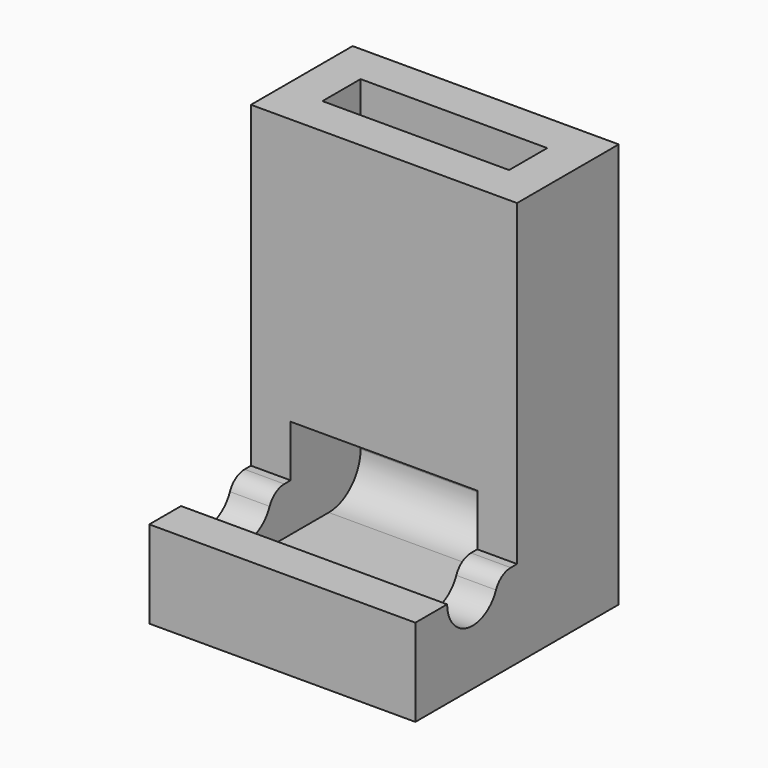
from build123d import *

# Parameters (mm, degrees)
F1_DEPTH  = 67
F2_W      = 47
F2_H      = 12
F3_DEPTH  = 92
F4_DEPTH  = 92
F5_W      = 47
F5_H      = 22
F6_DEPTH  = 12
F8_DEPTH  = 22
F9_R      = 9.99999
F11_DEPTH = 83
F12_R     = 5


# Not quite as in the source:
# - a fillet or chamfer is up to 0.001 mm smaller than in the source, because OpenCascade refuses the exact size


with BuildPart() as f1:
    # F0 (on Right) → F1 (new body)
    with BuildSketch(Plane.YZ):
        Polygon((0, 22), (0, 0), (64, 0), (64, 22), (64, 102), (32, 102), (32, 22), align=None)
    extrude(amount=-F1_DEPTH)

    # F2 (on face) → F3 (join)
    with BuildSketch(Plane.XY.offset(102)):
        with Locations((-33.5, 48)):
            Rectangle(F2_W, F2_H)
    extrude(amount=-F3_DEPTH)

    # F2 (on face) → F4 (cut)
    with BuildSketch(Plane.XY.offset(102)):
        with Locations((-33.5, 48)):
            Rectangle(F2_W, F2_H)
    extrude(amount=-F4_DEPTH, mode=Mode.SUBTRACT)

    # F5 (on face) → F6 (cut)
    with BuildSketch(Plane.XY.offset(22)):
        with Locations((-33.5, 21)):
            Rectangle(F5_W, F5_H)
    extrude(amount=-F6_DEPTH, mode=Mode.SUBTRACT)

    # F7 (on face) → F8 (cut)
    with BuildSketch(Plane.XZ.offset(-32)):
        Polygon((-57, 22), (-57, 10), (-10, 10), (-10, 22), (-10, 35), (-57, 35), align=None)
    extrude(amount=-F8_DEPTH, mode=Mode.SUBTRACT)

    # F9 (radius 10 in the source; OpenCascade refuses exactly that, so slightly less here)
    f9_edges = [f1.edges().sort_by_distance(p)[0] for p in [
        (-33.5, 54, 10),
        (-33.5, 42, 35),
    ]]
    fillet(f9_edges, radius=F9_R)

    # F10 (on face) → F11 (cut)
    with BuildSketch(Plane.YZ):
        with BuildLine():
            ThreePointArc((10, 22), (18, 14), (26, 22))
            Line((26, 22), (10, 22))
        make_face()
    extrude(amount=-F11_DEPTH, mode=Mode.SUBTRACT)

    # F12
    f12_edges = [f1.edges().sort_by_distance(p)[0] for p in [
        (-5, 26, 22),
        (-62, 26, 22),
    ]]
    fillet(f12_edges, radius=F12_R)


solid = f1.part
